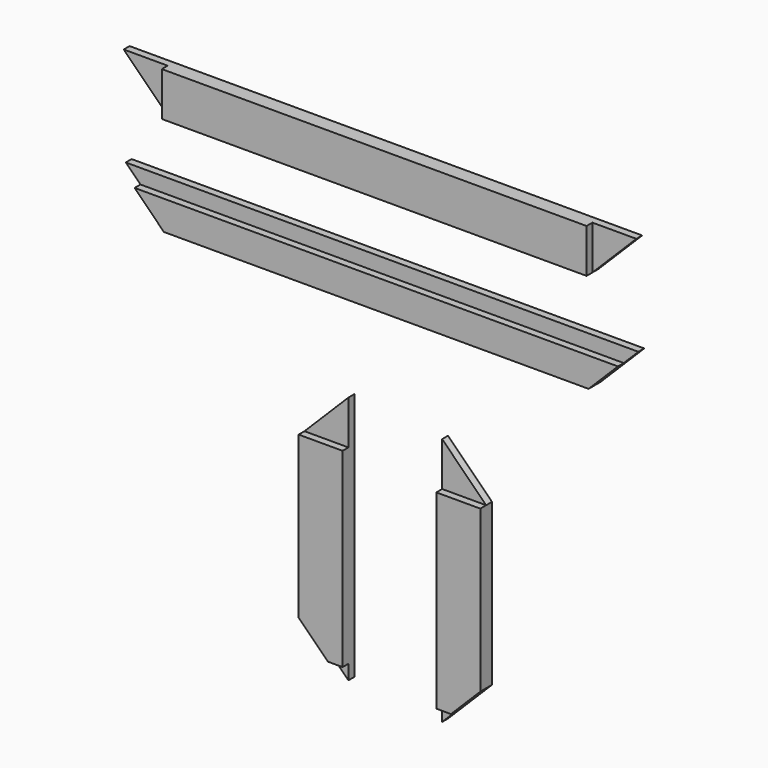
from build123d import *

# Parameters (mm, degrees)
F0_W       = 350
F0_H       = 30
F1_DEPTH   = 10
F0_W_2     = 30
F0_H_2     = 170
F2_W       = 30
F2_H       = 30
F3_DEPTH   = 5
F4_W       = 30
F4_H       = 30
F4_H_2     = 10
F5_DEPTH   = 5
F6_W       = 30
F6_H       = 30
F6_H_2     = 10
F7_DEPTH   = 5
F8_W       = 350
F8_H       = 30
F9_DEPTH   = 5
F10_W      = 350
F10_H      = 20
F11_DEPTH  = 5
F12_SIZE   = 29.99999
F12_2_SIZE = 29.99999
F12_3_SIZE = 29.99999
F12_4_SIZE = 29.99999


# Not quite as in the source:
# - a fillet or chamfer is up to 0.001 mm smaller than in the source, because OpenCascade refuses the exact size


with BuildPart() as f1:
    # F0 (on Front) → F1 (new body)
    with BuildSketch(Plane.XZ):
        with Locations((-21.6247046013, 106.3088514348)):
            Rectangle(F0_W, F0_H)
    extrude(amount=F1_DEPTH)

    # F2 (on face) → F3 (cut)
    with BuildSketch(Plane.XZ.offset(10)):
        with Locations((-181.6247046013, 106.3088514348)):
            Rectangle(F2_W, F2_H)
        with Locations((138.3752953987, 106.3088514348)):
            Rectangle(F2_W, F2_H)
    extrude(amount=-F3_DEPTH, mode=Mode.SUBTRACT)

    # F12 (size 30 in the source; OpenCascade refuses exactly that, so slightly less here)
    f12_edges = [f1.edges().sort_by_distance(p)[0] for p in [
        (-196.624705, -2.5, 91.308851),
        (153.375295, -2.5, 91.308851),
    ]]
    chamfer(f12_edges, length=F12_SIZE)


with BuildPart() as f1b:
    # F0 (on Front) → F1, piece 2 (new body)
    with BuildSketch(Plane.XZ):
        with Locations((-58.2107634842, -123.0070780963)):
            Rectangle(F0_W_2, F0_H_2)
    extrude(amount=F1_DEPTH)

    # F4 (on face) → F5 (cut)
    with BuildSketch(Plane.XZ.offset(10)):
        with Locations((-58.2107634842, -53.0070780963)):
            Rectangle(F4_W, F4_H)
        with Locations((-58.2107634842, -203.0070780963)):
            Rectangle(F4_W, F4_H_2)
    extrude(amount=-F5_DEPTH, mode=Mode.SUBTRACT)

    # F12#3 (size 30 in the source; OpenCascade refuses exactly that, so slightly less here)
    f12_3_edges = [f1b.edges().sort_by_distance(p)[0] for p in [
        (-73.210763, -2.5, -38.007078),
        (-73.210763, -2.5, -208.007078),
    ]]
    chamfer(f12_3_edges, length=F12_3_SIZE)


with BuildPart() as f1c:
    # F0 (on Front) → F1, piece 3 (new body)
    with BuildSketch(Plane.XZ):
        with Locations((35.80392465, -127.1743857861)):
            Rectangle(F0_W_2, F0_H_2)
    extrude(amount=F1_DEPTH)

    # F6 (on face) → F7 (cut)
    with BuildSketch(Plane.XZ.offset(10)):
        with Locations((35.80392465, -57.1743857861)):
            Rectangle(F6_W, F6_H)
        with Locations((35.80392465, -207.1743857861)):
            Rectangle(F6_W, F6_H_2)
    extrude(amount=-F7_DEPTH, mode=Mode.SUBTRACT)

    # F12#2 (size 30 in the source; OpenCascade refuses exactly that, so slightly less here)
    f12_2_edges = [f1c.edges().sort_by_distance(p)[0] for p in [
        (50.803925, -2.5, -42.174386),
        (50.803925, -2.5, -212.174386),
    ]]
    chamfer(f12_2_edges, length=F12_2_SIZE)


with BuildPart() as f9:
    # F8 (on Front) → F9 (new body)
    with BuildSketch(Plane.XZ):
        with Locations((-20.2150419354, 38.859708766)):
            Rectangle(F8_W, F8_H)
    extrude(amount=F9_DEPTH)

    # F10 (on face) → F11 (join)
    with BuildSketch(Plane.XZ.offset(5)):
        with Locations((-20.2150419354, 33.859708766)):
            Rectangle(F10_W, F10_H)
    extrude(amount=F11_DEPTH)

    # F12#4 (size 30 in the source; OpenCascade refuses exactly that, so slightly less here)
    f12_4_edges = [f9.edges().sort_by_distance(p)[0] for p in [
        (-195.215042, -5, 23.859709),
        (154.784958, -5, 23.859709),
    ]]
    chamfer(f12_4_edges, length=F12_4_SIZE)


solid = Compound([f1.part, f1b.part, f1c.part, f9.part])
